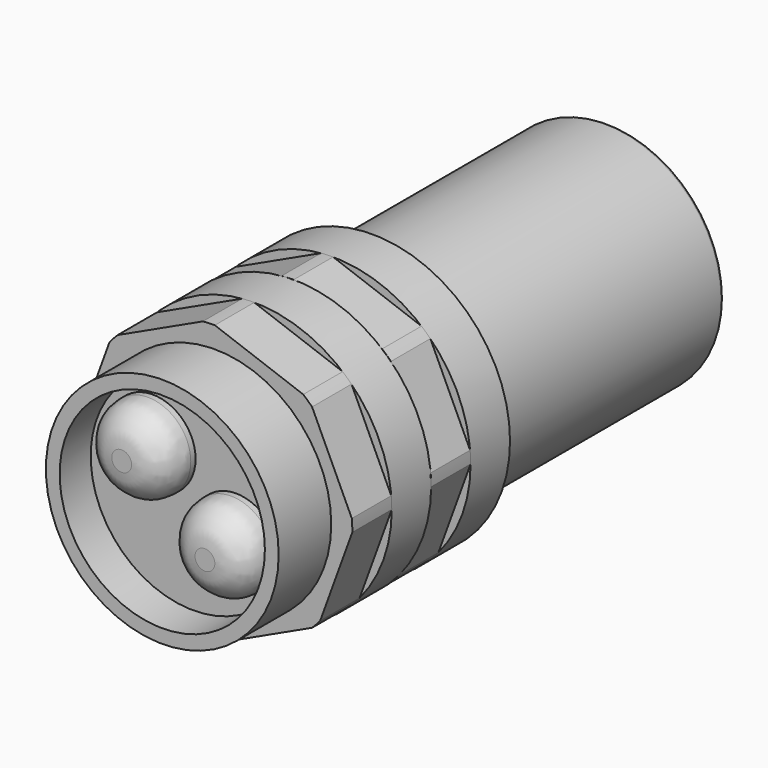
from build123d import *

# Parameters (mm, degrees)
F0_R             = 9
F1_DEPTH         = 43
F2_R             = 7.9338373334
F2_R_2           = 3.3064142063
F2_R_3           = 3.3078684587
F3_DEPTH         = 3
F4_DEPTH         = 0.005
F5_R             = 2.54
F6_R             = 0.254
F8_R             = 10.630598255
F9_DEPTH         = 3.81
F10_DEPTH        = 3.81
F11_DEPTH        = 3.81
F12_DEPTH        = 3.81
F14_DEPTH        = 3.81
F14_COPIES_COUNT = 8
F16_DEPTH        = 3.81
F16_COPIES_COUNT = 8


# Not quite as in the source:
# - a pattern or mirror of a feature is missing from the dataset's text; its kind, count and spacing are read off the source's solid


with BuildPart() as f1:
    # F0 (on Front) → F1 (new body)
    with BuildSketch(Plane.XZ):
        Circle(F0_R)
    extrude(amount=-F1_DEPTH)

    # F2 (on face) → F3 (cut)
    with BuildSketch(Plane.XZ):
        Circle(F2_R)
        with Locations((3.3013214234, -2.1994818862)):
            Circle(F2_R_2, mode=Mode.SUBTRACT)
        with Locations((-3.133161364, 2.4330523165)):
            Circle(F2_R_3, mode=Mode.SUBTRACT)
    extrude(amount=-F3_DEPTH, mode=Mode.SUBTRACT)

    # F4 (add): faces of the model
    f4_faces = [f1.faces().sort_by_distance(p)[0] for p in [
        (-3.133161364, 0, 2.4330523165),
        (3.3013214234, 0, -2.1994818862),
    ]]
    extrude(f4_faces, amount=F4_DEPTH)

    # F5
    f5_edges = [f1.edges().sort_by_distance(p)[0] for p in [
        (-6.44103, -0.005, 2.433052),
        (-0.005093, -0.005, -2.199482),
    ]]
    fillet(f5_edges, radius=F5_R)

    # F6
    f6_edges = [f1.edges().sort_by_distance(p)[0] for p in [
        (-9, 43, 0),
    ]]
    fillet(f6_edges, radius=F6_R)


with BuildPart() as f9:
    # F8 (on offset) → F9 (new body)
    with BuildSketch(Plane.XZ.offset(-5.08)):
        Circle(F8_R)
    extrude(amount=-F9_DEPTH)


with BuildPart() as f10:
    # F10 (new): a face of the model
    f10_faces = [f9.part.faces().sort_by_distance(p)[0] for p in [
        (0, 8.89, 0),
    ]]
    extrude(f10_faces, amount=F10_DEPTH)


with BuildPart() as f11:
    # F11 (new): a face of the model
    f11_faces = [f10.part.faces().sort_by_distance(p)[0] for p in [
        (0, 12.7, 0),
    ]]
    extrude(f11_faces, amount=F11_DEPTH)


with BuildPart() as f12:
    # F12 (new): a face of the model
    f12_faces = [f11.part.faces().sort_by_distance(p)[0] for p in [
        (0, 16.51, 0),
    ]]
    extrude(f12_faces, amount=F12_DEPTH)


with BuildPart() as f9_1:
    add(f9.part)

    # F13 (on face) → F14 (cut)
    with BuildSketch(Plane.XZ.offset(-5.08)):
        with BuildLine():
            ThreePointArc((6.8332168419, 8.1435107203), (3.6358787388, 9.9894947348), (0, 10.630598255))
            Line((0, 10.630598255), (6.8332168419, 8.1435107203))
        make_face()
    f14 = extrude(amount=-F14_DEPTH, mode=Mode.SUBTRACT)

    # F14_copies: F14 ×8 about axis
    f14_copies_axis = Axis((0, 0, 0), (0, 1, 0))
    for i in range(1, F14_COPIES_COUNT):
        add(f14.rotate(f14_copies_axis, i * 360 / F14_COPIES_COUNT), mode=Mode.SUBTRACT)


with BuildPart() as f11_1:
    add(f11.part)

    # F15 (on face) → F16 (cut)
    with BuildSketch(Plane.XZ.offset(-12.7)):
        with BuildLine():
            Line((0, 10.630598255), (6.8332168419, 8.1435107203))
            ThreePointArc((6.8332168419, 8.1435107203), (3.6358787388, 9.9894947348), (0, 10.630598255))
        make_face()
    f16 = extrude(amount=-F16_DEPTH, mode=Mode.SUBTRACT)

    # F16_copies: F16 ×8 about axis
    f16_copies_axis = Axis((0, 0, 0), (0, 1, 0))
    for i in range(1, F16_COPIES_COUNT):
        add(f16.rotate(f16_copies_axis, i * 360 / F16_COPIES_COUNT), mode=Mode.SUBTRACT)


solid = Compound([f1.part, f10.part, f12.part, f9_1.part, f11_1.part])
